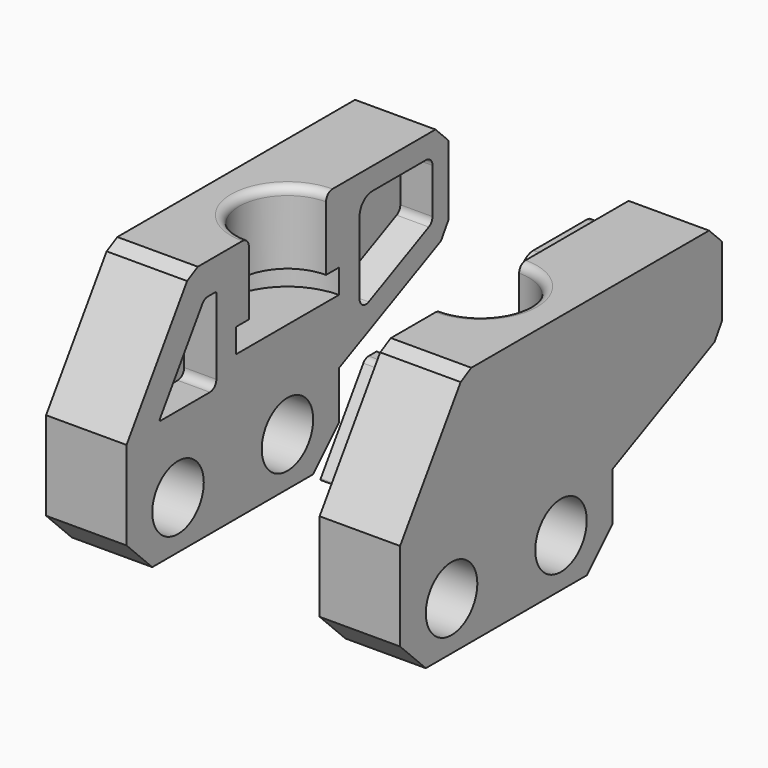
from build123d import *

# Parameters (mm, degrees)
F1_DEPTH     = 5
F3_DEPTH     = 6
F4_DEPTH     = 4.5
F5_R         = 0.5
F7_DEPTH     = 2
F6_R         = 2
F8_DEPTH     = 25
F9_SIZE      = 2
F10_T1_DEPTH = 10.1433659759
F10_T3_DEPTH = 8.3436121046
F10_T5_DEPTH = 7.853814506
F15_DEPTH    = 4


# Not quite as in the source:
# - a fillet or chamfer that OpenCascade refuses, or shapes differently, is made with other operations: its cross-section is extruded or revolved along the edge and cut away or added


with BuildPart() as f1:
    # F0 (on Right) → F1 (new body)
    with BuildSketch(Plane.YZ):
        Polygon((0, 6.6470588235), (0, 15), (-15, 15), (-20, 7.5), (-20, 0), (-15, 0), (-3.5, 0), (-3.5, 5), align=None)
        Polygon((5, 15), (0, 15), (0, 6.6470588235), (5, 9), align=None)
    extrude(amount=-F1_DEPTH)

    # F2 (on face) → F3 (cut)
    with BuildSketch(Plane.XY.offset(15)):
        with BuildLine():
            Line((0, -4.5), (0, -3.5))
            ThreePointArc((0, -3.5), (-4, -7.5), (0, -11.5))
            Line((0, -11.5), (0, -10.5))
            ThreePointArc((0, -10.5), (-3, -7.5), (0, -4.5))
        make_face()
        with BuildLine():
            Line((0, -10.5), (0, -4.5))
            ThreePointArc((0, -4.5), (-3, -7.5), (0, -10.5))
        make_face()
    extrude(amount=-F3_DEPTH, mode=Mode.SUBTRACT)

    # F2 (on face) → F4 (join)
    with BuildSketch(Plane.XY.offset(15)):
        with BuildLine():
            Line((0, -4.5), (0, -3.5))
            ThreePointArc((0, -3.5), (-4, -7.5), (0, -11.5))
            Line((0, -11.5), (0, -10.5))
            ThreePointArc((0, -10.5), (-3, -7.5), (0, -4.5))
        make_face()
    extrude(amount=-F4_DEPTH)

    # F5
    f5_edges = [f1.edges().sort_by_distance(p)[0] for p in [
        (-3, -7.5, 15),
    ]]
    fillet(f5_edges, radius=F5_R)

    # F6 (on face) → F7 (cut)
    with BuildSketch(Plane.YZ):
        with BuildLine():
            ThreePointArc((-13.5242807064, 7.7500004351), (-13.1707273158, 7.8964470445), (-13.0242807064, 8.2500004351))
            Line((-13.0242807064, 8.2500004351), (-13.0242807064, 12.9757192936))
            ThreePointArc((-13.0242807064, 12.9757192936), (-13.0460368942, 13.0282433771), (-13.0985609777, 13.0499995649))
            Line((-13.0985609777, 13.0499995649), (-13.6887995588, 13.0499995649))
            ThreePointArc((-13.6887995588, 13.0499995649), (-13.9247285216, 12.9908368643), (-14.104824706, 12.827349663))
            Line((-14.104824706, 12.827349663), (-17.4127351563, 7.8654839875))
            ThreePointArc((-17.4127351563, 7.8654839875), (-17.4164212631, 7.7892309717), (-17.3509302347, 7.7500004351))
            Line((-17.3509302347, 7.7500004351), (-13.5242807064, 7.7500004351))
        make_face()
        with BuildLine():
            Line((3.7674111893, 10.3282596764), (3.7674111893, 13.1287492136))
            ThreePointArc((3.7674111893, 13.1287492136), (3.6209645799, 13.4823026042), (3.2674111893, 13.6287492136))
            Line((3.2674111893, 13.6287492136), (-0.9, 13.6287492136))
            ThreePointArc((-0.9, 13.6287492136), (-1.6071067812, 13.3358559948), (-1.9, 12.6287492136))
            Line((-1.9, 12.6287492136), (-1.9, 8.1318308814))
            ThreePointArc((-1.9, 8.1318308814), (-1.6679092579, 7.7096642916), (-1.1871014818, 7.6794215303))
            Line((-1.1871014818, 7.6794215303), (3.4803097074, 9.8758503253))
            ThreePointArc((3.4803097074, 9.8758503253), (3.6895777791, 10.0603504185), (3.7674111893, 10.3282596764))
        make_face()
    extrude(amount=-F7_DEPTH, mode=Mode.SUBTRACT)

    # F6 (on face) → F8 (cut)
    with BuildSketch(Plane.YZ):
        with Locations((-16, 3)):
            Circle(F6_R)
        with Locations((-7.5, 3)):
            Circle(F6_R)
    extrude(amount=-F8_DEPTH, mode=Mode.SUBTRACT)

    # F9
    f9_edges = [f1.edges().sort_by_distance(p)[0] for p in [
        (-2.5, -20, 0),
        (-2.5, -3.5, 0),
    ]]
    chamfer(f9_edges, length=F9_SIZE)

    # F10: chamfer of 1 on 3 edges, made by hand

    # F10_s2 → F10_t1 (cut)
    with BuildSketch(Plane.YZ.offset(-7.571682988)):
        Polygon((4, 15), (5, 14), (5, 15), align=None)
    extrude(amount=F10_T1_DEPTH, mode=Mode.SUBTRACT)

    # F10_s4 → F10_t3 (cut)
    with BuildSketch(Plane.YZ.offset(-6.6718060523)):
        Polygon((4.4257970363, 8.7297868406), (5, 9.6346055428), (5, 9), align=None)
    extrude(amount=F10_T3_DEPTH, mode=Mode.SUBTRACT)

    # F10_s6 → F10_t5 (cut)
    with BuildSketch(Plane.YZ.offset(-6.426907253)):
        Polygon((-15.2968665358, 14.5547001962), (-14.4648162415, 15), (-15, 15), align=None)
    extrude(amount=F10_T5_DEPTH, mode=Mode.SUBTRACT)


with BuildPart() as f14_1:
    # F14: instance of F1
    add(f1.part.mirror(Plane.YZ.offset(6)))

    # F15 (add): faces of the model
    f15_faces = [f14_1.faces().sort_by_distance(p)[0] for p in [
        (14, 0.7023595879, 11.0891845918),
        (14, -14.5715468985, 9.8270536303),
    ]]
    extrude(f15_faces, amount=F15_DEPTH)


solid = Compound([f1.part, f14_1.part])
